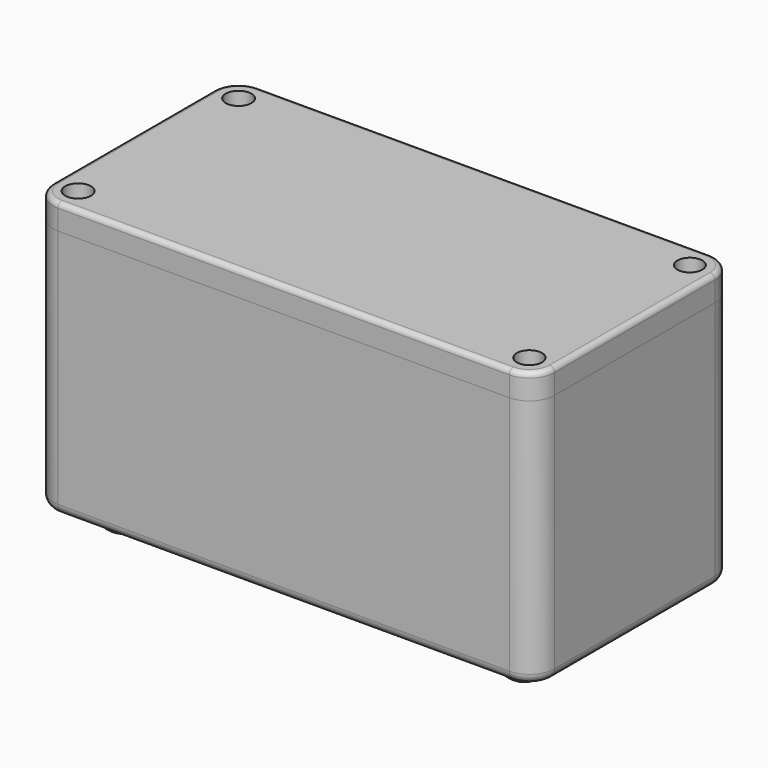
from build123d import *

# Parameters (mm, degrees)
F0_W      = 100
F0_H      = 50
F1_DEPTH  = 50
F2_W      = 90
F2_H      = 40.0000010431
F3_DEPTH  = 45
F4_W      = 5
F4_H      = 5
F5_DEPTH  = 45
F7_D      = 5
F7_DEPTH  = 12
F7_TIP    = 1.5021515476
F8_R      = 5
F9_R      = 2.5769210798
F9_R_2    = 2.5224628813
F9_R_3    = 2.5607989108
F9_R_4    = 2.4914116102
F10_DEPTH = 5
F11_R     = 5
F12_DEPTH = 5
F13_R     = 4.99999
F14_R     = 2
F15_R     = 1


# Not quite as in the source:
# - a fillet or chamfer is up to 0.001 mm smaller than in the source, because OpenCascade refuses the exact size


with BuildPart() as f1:
    # F0 (on Top) → F1 (new body)
    with BuildSketch(Plane.XY):
        with Locations((50, 25)):
            Rectangle(F0_W, F0_H)
    extrude(amount=F1_DEPTH)

    # F2 (on face) → F3 (cut)
    with BuildSketch(Plane.XY.offset(50)):
        with Locations((50, 25.0000005215)):
            Rectangle(F2_W, F2_H)
    extrude(amount=-F3_DEPTH, mode=Mode.SUBTRACT)

    # F4 (on face) → F5 (join)
    with BuildSketch(Plane.XY.offset(5)):
        with Locations((7.5, 42.5000010431)):
            Rectangle(F4_W, F4_H)
        with Locations((7.5, 7.5)):
            Rectangle(F4_W, F4_H)
        with Locations((92.5, 42.5000010431)):
            Rectangle(F4_W, F4_H)
        with Locations((92.5, 7.5)):
            Rectangle(F4_W, F4_H)
    extrude(amount=F5_DEPTH)

    # F7
    with Locations(Plane.XY.offset(50)):
        with Locations((5, 45.0000010431), (5, 5), (95, 5), (95, 45.0000010431)):
            Hole(F7_D / 2, depth=F7_DEPTH)
            with Locations((0, 0, -(F7_DEPTH + F7_TIP / 2))):  # 118° drill point
                Cone(0, F7_D / 2, F7_TIP, mode=Mode.SUBTRACT)

    # F8
    f8_edges = [f1.edges().sort_by_distance(p)[0] for p in [
        (0, 0, 25),
        (0, 50, 25),
        (100, 50, 25),
        (100, 0, 25),
    ]]
    fillet(f8_edges, radius=F8_R)

    # F11 (on face) → F12 (join)
    with BuildSketch(Plane(origin=(0, 0, 0), x_dir=(1, 0, 0), z_dir=(0, 0, -1))):
        with Locations((10, -10)):
            Circle(F11_R)
        with Locations((90, -10)):
            Circle(F11_R)
        with Locations((90, -40)):
            Circle(F11_R)
        with Locations((10, -40)):
            Circle(F11_R)
    extrude(amount=F12_DEPTH)

    # F13 (radius 5 in the source; OpenCascade refuses exactly that, so slightly less here)
    f13_edges = [f1.edges().sort_by_distance(p)[0] for p in [
        (5, 10, -5),
        (5, 40, -5),
        (85, 10, -5),
        (85, 40, -5),
    ]]
    fillet(f13_edges, radius=F13_R)

    # F14
    f14_edges = [f1.edges().sort_by_distance(p)[0] for p in [
        (0, 25, 0),
    ]]
    fillet(f14_edges, radius=F14_R)


with BuildPart() as f10:
    # F9 (on face) → F10 (new body)
    with BuildSketch(Plane.XY.offset(50)):
        with BuildLine():
            Line((95, 50), (5, 50))
            ThreePointArc((5, 50), (1.4644660941, 48.5355339059), (0, 45))
            Line((0, 45), (0, 5))
            ThreePointArc((0, 5), (1.4644660941, 1.4644660941), (5, 0))
            Line((5, 0), (95, 0))
            ThreePointArc((95, 0), (98.5355339059, 1.4644660941), (100, 5))
            Line((100, 5), (100, 45))
            ThreePointArc((100, 45), (98.5355339059, 48.5355339059), (95, 50))
        make_face()
        with Locations((5, 5)):
            Circle(F9_R, mode=Mode.SUBTRACT)
        with Locations((95, 5)):
            Circle(F9_R_2, mode=Mode.SUBTRACT)
        with Locations((5, 45.0000010431)):
            Circle(F9_R_3, mode=Mode.SUBTRACT)
        with Locations((95, 45.0000010431)):
            Circle(F9_R_4, mode=Mode.SUBTRACT)
    extrude(amount=F10_DEPTH)

    # F15
    f15_edges = [f10.edges().sort_by_distance(p)[0] for p in [
        (50, 50, 55),
    ]]
    fillet(f15_edges, radius=F15_R)


solid = Compound([f1.part, f10.part])
